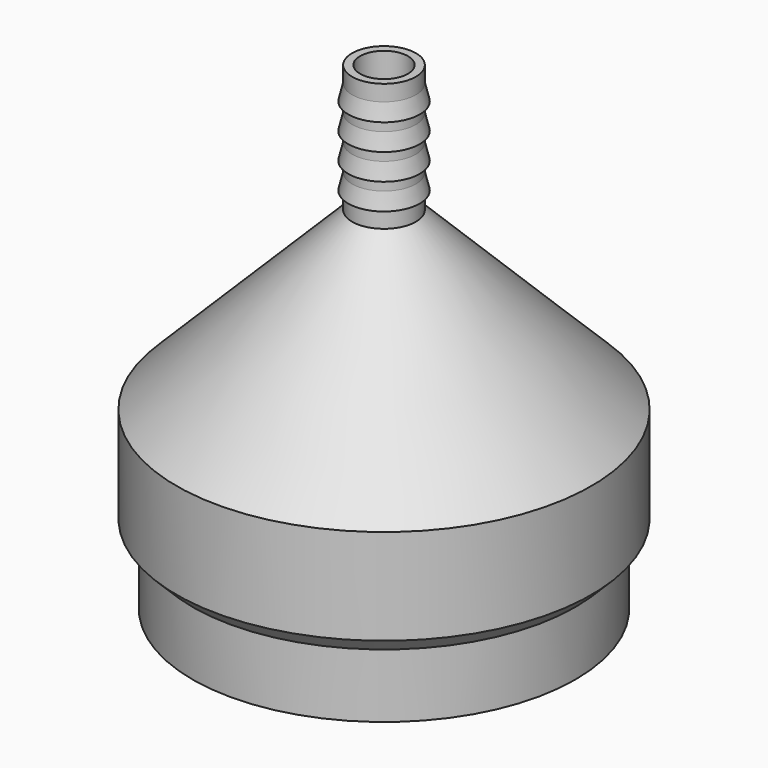
from build123d import *

# Parameters (mm, degrees)
F3_DEPTH = 12.7


with BuildPart() as f1:
    # F0 (on Front) → F1 (revolve)
    with BuildSketch(Plane.XZ):
        Polygon((-38.1, 0), (-34.925, 0), (-34.925, 19.05), (-38.1, 19.05), (-38.1, 34.925), (-4.7625, 68.2625), (-4.7625, 95.25), (-6.35, 95.25), (-6.35, 92.075), (-7.112, 88.9), (-6.35, 88.9), (-6.35, 86.868), (-7.112, 83.693), (-6.35, 83.693), (-6.35, 81.661), (-7.112, 78.486), (-6.35, 78.486), (-6.35, 76.454), (-7.112, 73.279), (-6.35, 73.279), (-6.35, 69.85), (-41.275, 34.925), (-41.275, 15.875), (-38.1, 12.7), align=None)
    revolve(axis=Axis((0, 0, 50.8), (0, 0, 1)))


with BuildPart() as f3:
    # F2 (on Top) → F3 (new body)
    with BuildSketch(Plane.XY):
        with BuildLine():
            Line((-3.1749960745, -28.3980637531), (-3.1749960745, -34.7751258129))
            ThreePointArc((-3.1749960745, -34.7751258129), (2.24367e-05, -34.9249723343), (3.1750395166, -34.7750954884))
            Line((3.1750395166, -34.7750954884), (3.1750409639, -28.3980587343))
            ThreePointArc((3.1750409639, -28.3980587343), (10.9352255737, -26.3998383831), (17.8354455442, -22.3254900783))
            Line((17.8354455442, -22.3254900783), (22.3460920856, -26.8361386672))
            ThreePointArc((22.3460920856, -26.8361386672), (24.695725028, -24.6956852351), (26.8361753226, -22.3460494346))
            Line((26.8361753226, -22.3460494346), (22.3255262075, -17.8354003195))
            ThreePointArc((22.3255262075, -17.8354003195), (26.3998576023, -10.9351791745), (28.3980634632, -3.1749986674))
            Line((28.3980634632, -3.1749986674), (34.7751405906, -3.1749986674))
            ThreePointArc((34.7751405906, -3.1749986674), (34.925, 1.3605e-06), (34.7751394094, 3.1750013326))
            Line((34.7751394094, 3.1750013326), (28.3980631653, 3.1750013326))
            ThreePointArc((28.3980631653, 3.1750013326), (26.3998585218, 10.9351769545), (22.3255308809, 17.8353944696))
            Line((22.3255308809, 17.8353944696), (26.8361885113, 22.3460520999))
            ThreePointArc((26.8361885113, 22.3460520999), (24.6957050465, 24.6957139393), (22.3460476901, 26.8362023251))
            Line((22.3460476901, 26.8362023251), (17.835384339, 22.325538974))
            ThreePointArc((17.835384339, 22.325538974), (10.9351680084, 26.3998622274), (3.1749949722, 28.3980638764))
            Line((3.1749949722, 28.3980638764), (3.1749949722, 34.7751420859))
            ThreePointArc((3.1749949722, 34.7751420859), (1.3068e-06, 34.9250056515), (-3.17499275, 34.7751503786))
            Line((-3.17499275, 34.7751503786), (-3.17499275, 28.3980641248))
            ThreePointArc((-3.17499275, 28.3980641248), (-10.9351754232, 26.3998591561), (-17.8353986269, 22.3255275597))
            Line((-17.8353986269, 22.3255275597), (-22.3460490284, 26.8361779611))
            ThreePointArc((-22.3460490284, 26.8361779611), (-24.6756495106, 24.6756879964), (-26.8361394753, 22.3460875142))
            Line((-26.8361394753, 22.3460875142), (-22.3254933767, 17.8354414156))
            ThreePointArc((-22.3254933767, 17.8354414156), (-26.3998402061, 10.9352211725), (-28.3980592058, 3.1750367469))
            Line((-28.3980592058, 3.1750367469), (-34.7751006475, 3.1750367469))
            ThreePointArc((-34.7751006475, 3.1750367469), (-34.9249999999, 1.72484e-05), (-34.7751458819, -3.1750043854))
            Line((-34.7751458819, -3.1750043854), (-28.3980628239, -3.1750043854))
            ThreePointArc((-28.3980628239, -3.1750043854), (-26.3998554001, -10.935184491), (-22.3255226152, -17.8354048162))
            Line((-22.3255226152, -17.8354048162), (-26.8361646407, -22.3460468418))
            ThreePointArc((-26.8361646407, -22.3460468418), (-24.6956947976, -24.6956947976), (-22.3460468418, -26.8361646407))
            Line((-22.3460468418, -26.8361646407), (-17.8354048162, -22.3255226152))
            ThreePointArc((-17.8354048162, -22.3255226152), (-10.9351806279, -26.3998570003), (-3.1749960745, -28.3980637531))
        make_face()
    extrude(amount=F3_DEPTH)


solid = Compound([f1.part, f3.part])
